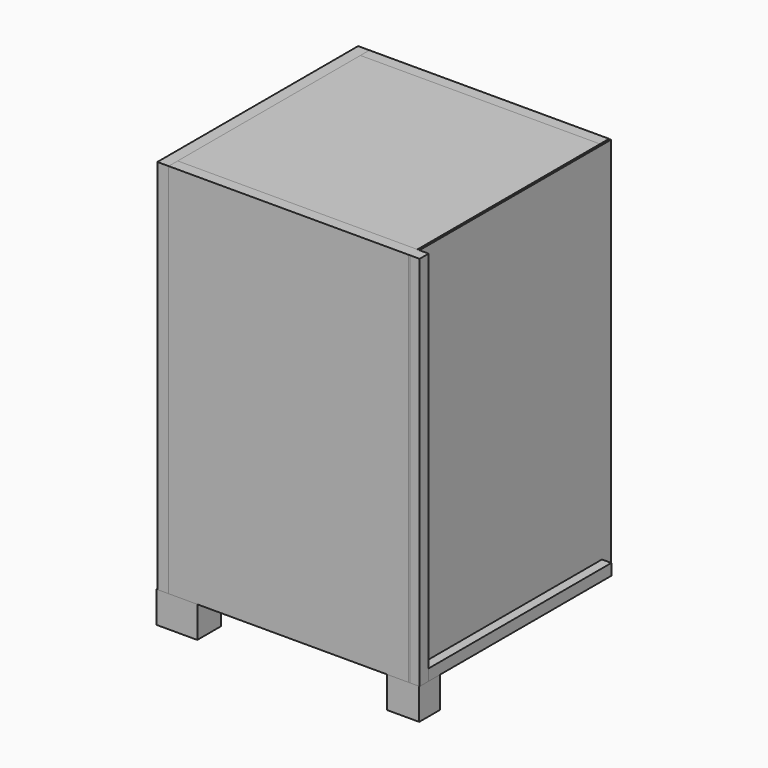
from build123d import *

# Parameters (mm, degrees)
F0_W      = 200
F0_H      = 300
F1_DEPTH  = 9
F3_DEPTH  = 12
F5_DEPTH  = 182
F7_DEPTH  = 12
F8_W      = 15.0606025722
F8_H      = 50.1502417028
F9_DEPTH  = 5
F10_W     = 191
F10_H     = 9
F11_DEPTH = 182
F12_W     = 200
F12_H     = 9
F13_DEPTH = 182
F14_W     = 191
F14_H     = 300
F16_DEPTH = 9
F17_W     = 200
F17_H     = 299.8089425825
F18_DEPTH = 1.5
F19_W     = 200
F19_H     = 300
F20_DEPTH = 9
F21_R     = 38.194679826
F22_DEPTH = 30
F23_W     = 32.3943905532
F23_H     = 23.6132256687
F24_DEPTH = 25
F25_W     = 25.5955606699
F25_H     = 20.9072008729
F26_DEPTH = 25
F27_W     = 26.3972375542
F27_H     = 19.920361042
F28_DEPTH = 25


# Not quite as in the source:
# - a feature names something its author has since deleted; it is built from what else it names


with BuildPart() as f1:
    # F0 (on Front) → F1 (new body)
    with BuildSketch(Plane.XZ):
        with Locations((100, 150)):
            Rectangle(F0_W, F0_H)
    extrude(amount=-F1_DEPTH)


with BuildPart() as f3:
    # F2 (on face) → F3 (new body)
    with BuildSketch(Plane(origin=(0, 9, 0), x_dir=(-1, 0, 0), z_dir=(0, 1, 0))):
        Polygon((-161.8147794008, 157.7074974775), (-191, 178.9015382528), (-191, 138.5981291533), align=None)
    extrude(amount=F3_DEPTH)


with BuildPart() as f5:
    # F4 (on face) → F5 (new body)
    with BuildSketch(Plane(origin=(0, 9, 0), x_dir=(-1, 0, 0), z_dir=(0, 1, 0))):
        Polygon((-191, 178.9015382528), (-161.8147794008, 157.7074974775), (-156.8773534762, 164.5065721009), (-186.0625740754, 185.7006128762), align=None)
    extrude(amount=F5_DEPTH)


with BuildPart() as f7:
    # F6 (on face) → F7 (new body)
    with BuildSketch(Plane(origin=(0, 191, 0), x_dir=(-1, 0, 0), z_dir=(0, 1, 0))):
        Polygon((-161.8147794008, 157.7074974775), (-191, 178.9015382528), (-191, 138.597920537), align=None)
    extrude(amount=-F7_DEPTH)


with BuildPart() as f9:
    # F8 (on face) → F9 (new body)
    with BuildSketch(Plane(origin=(-24.0503636645, 0, 33.1185155525), x_dir=(0.8091522816, 0, 0.5875990004), z_dir=(-0.5875990004, 0, 0.8091522816))):
        with Locations((231.1318670975, 86.4051077515)):
            Rectangle(F8_W, F8_H)
    extrude(amount=F9_DEPTH)


with BuildPart() as f11:
    # F10 (on face) → F11 (new body)
    with BuildSketch(Plane(origin=(0, 9, 0), x_dir=(-1, 0, 0), z_dir=(0, 1, 0))):
        with Locations((-95.5, 295.5)):
            Rectangle(F10_W, F10_H)
    extrude(amount=F11_DEPTH)


with BuildPart() as f13:
    # F12 (on face) → F13 (new body)
    with BuildSketch(Plane(origin=(0, 9, 0), x_dir=(-1, 0, 0), z_dir=(0, 1, 0))):
        with Locations((-100, 4.5)):
            Rectangle(F12_W, F12_H)
    extrude(amount=F13_DEPTH)


with BuildPart() as f16:
    # F14 (on face) → F16 (new body)
    with BuildSketch(Plane(origin=(0, 191, 0), x_dir=(-1, 0, 0), z_dir=(0, 1, 0))):
        with Locations((-95.5, 150)):
            Rectangle(F14_W, F14_H)
    extrude(amount=F16_DEPTH)


with BuildPart() as f18:
    # F17 (on face) → F18 (new body)
    with BuildSketch(Plane.YZ.offset(191)):
        with Locations((100, 149.9044712912)):
            Rectangle(F17_W, F17_H)
    extrude(amount=F18_DEPTH)


with BuildPart() as f20:
    # F19 (on face) → F20 (new body)
    with BuildSketch(Plane(origin=(0, 0, 0), x_dir=(0, -1, 0), z_dir=(-1, 0, 0))):
        with Locations((-100, 150)):
            Rectangle(F19_W, F19_H)
    extrude(amount=F20_DEPTH)

    # F21 (on face) → F22 (cut)
    with BuildSketch(Plane(origin=(-9, 0, 0), x_dir=(0, -1, 0), z_dir=(-1, 0, 0))):
        with Locations((-119.2174553871, 83.0505564809)):
            Circle(F21_R)
    extrude(amount=-F22_DEPTH, mode=Mode.SUBTRACT)


with BuildPart() as f24:
    # F23 (on face) → F24 (new body)
    with BuildSketch(Plane(origin=(0, 0, 0), x_dir=(1, 0, 0), z_dir=(0, 0, -1))):
        with Locations((6.6161714494, -11.8066128343)):
            Rectangle(F23_W, F23_H)
    extrude(amount=F24_DEPTH)


with BuildPart() as f26:
    # F25 (on face) → F26 (new body)
    with BuildSketch(Plane(origin=(0, 0, 0), x_dir=(1, 0, 0), z_dir=(0, 0, -1))):
        with Locations((186.878465116, -10.4536004364)):
            Rectangle(F25_W, F25_H)
    extrude(amount=F26_DEPTH)


with BuildPart() as f28:
    # F27 (on face) → F28 (new body)
    with BuildSketch(Plane(origin=(0, 0, 0), x_dir=(1, 0, 0), z_dir=(0, 0, -1))):
        with Locations((4.1986187771, -190.039819479)):
            Rectangle(F27_W, F27_H)
    extrude(amount=F28_DEPTH)


solid = Compound([f1.part, f3.part, f5.part, f7.part, f9.part, f11.part, f13.part, f16.part, f18.part, f20.part, f24.part, f26.part, f28.part])
